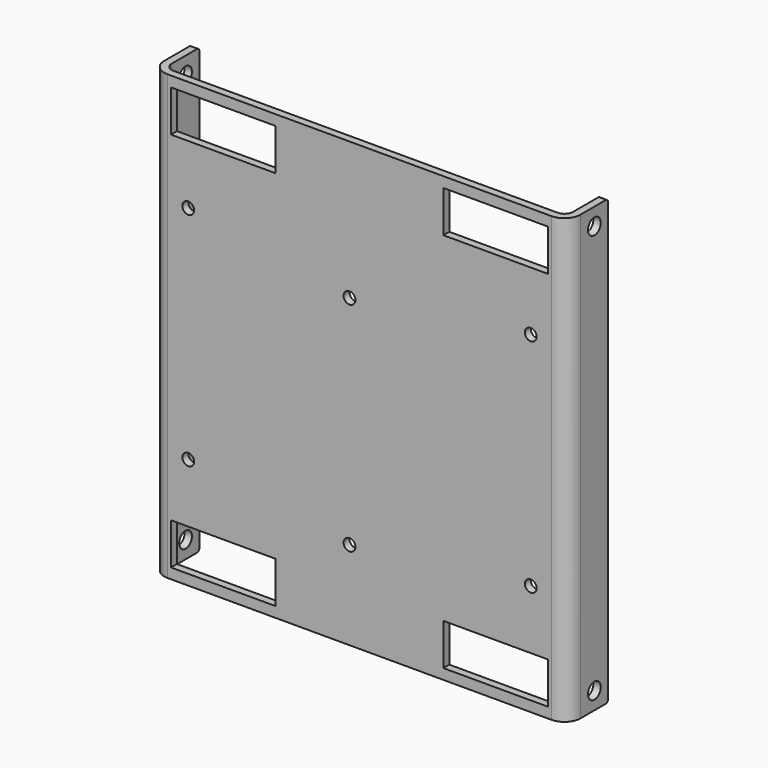
from build123d import *

# Parameters (mm, degrees)
F1_DEPTH  = 101.6
F2_R      = 3.69316
F3_R      = 1.98374
F4_W      = 24
F4_H      = 9.5329248
F4_R      = 1.35255
F5_DEPTH  = 1.70942
F6_R      = 1.8288
F7_DEPTH  = 95.37192
F8_R      = 0.762
F9_R      = 1.35255
F10_DEPTH = 1.70942


with BuildPart() as f1:
    # F0 (on Top) → F1 (new body)
    with BuildSketch(Plane.XY):
        Polygon((0, 9.92124), (0, 0), (-91.95308, 0), (-91.95308, 9.92124), (-93.6625, 9.92124), (-93.6625, -1.70942), (1.70942, -1.70942), (1.70942, 9.92124), align=None)
    extrude(amount=F1_DEPTH)

    # F2
    f2_edges = [f1.edges().sort_by_distance(p)[0] for p in [
        (1.70942, -1.70942, 50.8),
        (-93.6625, -1.70942, 50.8),
    ]]
    fillet(f2_edges, radius=F2_R)

    # F3
    f3_edges = [f1.edges().sort_by_distance(p)[0] for p in [
        (0, 0, 50.8),
        (-91.95308, 0, 50.8),
    ]]
    fillet(f3_edges, radius=F3_R)

    # F4 (on face) → F5 (cut, through all)
    with BuildSketch(Plane(origin=(0, 0, 0), x_dir=(-1, 0, 0), z_dir=(0, 1, 0))):
        with Locations((77.17559, 94.4522876)):
            Rectangle(F4_W, F4_H)
        with Locations((77.17559, 7.1477124)):
            Rectangle(F4_W, F4_H)
        with Locations((14.77749, 7.1477124)):
            Rectangle(F4_W, F4_H)
        with Locations((14.77749, 94.4522876)):
            Rectangle(F4_W, F4_H)
        with Locations((85.20684, 76.1477196107)):
            Circle(F4_R)
        with Locations((85.20684, 25.4522803893)):
            Circle(F4_R)
        with Locations((6.74624, 25.4522803893)):
            Circle(F4_R)
        with Locations((6.74624, 76.1477196107)):
            Circle(F4_R)
    extrude(amount=-F5_DEPTH, mode=Mode.SUBTRACT)

    # F6 (on face) → F7 (cut, through all)
    with BuildSketch(Plane.YZ.offset(1.70942)):
        with Locations((5.95249, 97.63125)):
            Circle(F6_R)
        with Locations((5.95249, 3.96875)):
            Circle(F6_R)
    extrude(amount=-F7_DEPTH, mode=Mode.SUBTRACT)

    # F8
    f8_edges = [f1.edges().sort_by_distance(p)[0] for p in [
        (-92.80779, 9.92124, 101.6),
        (-92.80779, 9.92124, 0),
        (0.85471, 9.92124, 0),
        (0.85471, 9.92124, 101.6),
    ]]
    fillet(f8_edges, radius=F8_R)

    # F9 (on face) → F10 (cut, through all)
    with BuildSketch(Plane(origin=(0, 0, 0), x_dir=(-1, 0, 0), z_dir=(0, 1, 0))):
        with Locations((48.26635, 70.0399442418)):
            Circle(F9_R)
        with Locations((48.26635, 20.2559442418)):
            Circle(F9_R)
    extrude(amount=-F10_DEPTH, mode=Mode.SUBTRACT)


solid = f1.part
